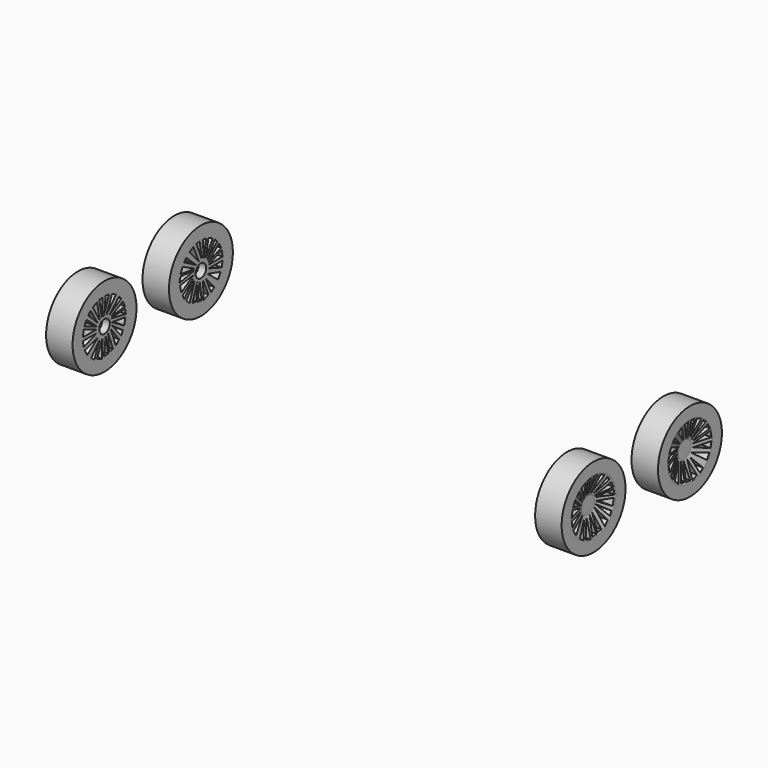
from build123d import *

# Parameters (mm, degrees)
F3_DEPTH = 54.356
F5_START = -2.0828
F4_R     = 1.016
F5_DEPTH = 5.588


# Not quite as in the source:
# - a feature names something its author has since deleted; it is built from what else it names


with BuildPart() as f1:
    # F0 (on Top) → F1 (revolve)
    with BuildSketch(Plane.XY):
        Polygon((-38.7761598104, 10.5307940394), (-38.7761598104, 9.2558898032), (-35.5391725898, 9.2558898032), (-35.5391725898, 15.3969740495), (-39.609067142, 15.3969740495), (-39.609067142, 13.5389780626), align=None)
    revolve(axis=Axis((-37.1576662001, 9.2558898032, 0), (1, 0, 0)))

    # F2 (on Right) → F3 (cut)
    with BuildSketch(Plane.YZ):
        Polygon((10.4703787739, -0.9244092506), (12.5581930749, -2.5232885566), (13.0646565989, -1.6865519105), align=None)
        Polygon((10.7676169888, -0.3009043154), (13.2498589973, -1.1950938976), (13.4170880637, -0.3009043154), align=None)
        Polygon((10.7827322258, 0.2167291751), (13.4224200405, 0.2167291751), (13.2498589973, 1.1950938976), align=None)
        Polygon((10.6890620408, 0.55644517), (13.1332652272, 1.5257193069), (12.7097717953, 2.3165763491), align=None)
        Polygon((11.9163488444, 3.1771167458), (10.4901476553, 0.8995587363), (12.3804111502, 2.7352948513), align=None)
        Polygon((11.4917309209, 3.4794998925), (10.6890620408, 3.8635174401), (10.1889797433, 1.1895302548), align=None)
        Polygon((9.647954578, 4.082242185), (9.7795484241, 1.3955574327), (10.2642306786, 3.9871991361), align=None)
        Polygon((8.386955188, 3.9871991361), (9.4131707997, 1.4628515054), (9.0197490168, 4.082242185), align=None)
        Polygon((7.0658904336, 3.4087700224), (8.8881551707, 1.3955574327), (7.823212836, 3.8054345011), align=None)
        Polygon((6.0489947183, 2.4439876807), (8.386955188, 1.1178608331), (6.4443791376, 2.9007429328), align=None)
        Polygon((5.3209666594, 1.1178608331), (8.0941571054, 0.7806299389), (5.7344314769, 1.9512906421), align=None)
        Polygon((5.156467886, 0), (7.978641554, 0.55644517), (5.3209666594, 0.8124744198), align=None)
        Polygon((5.4919943851, -1.4154481401), (7.8688514455, 0), (5.2583602836, -0.3920851117), align=None)
        Polygon((6.0489947183, -2.5315452176), (7.9222940422, -0.3920851117), (5.7344314769, -1.9512906421), align=None)
        Polygon((7.0658904336, -3.5198394674), (8.0941571054, -0.7806299389), (6.4443791376, -2.9007429328), align=None)
        Polygon((8.386955188, -3.7943273253), (8.5564610454, -1.2417284927), (7.6257726915, -3.7209981969), align=None)
        Polygon((9.4131707997, -4.0348388196), (9.0197490168, -1.4154481401), (8.5564610454, -3.952306996), align=None)
        Polygon((10.6991987211, -3.7943273253), (9.647954578, -1.4154481401), (9.7795484241, -4.1681900535), align=None)
        Polygon((11.8202538041, -3.2528705592), (10.1889797433, -1.4154481401), (11.2078192072, -3.7209981969), align=None)
    extrude(amount=-F3_DEPTH, mode=Mode.SUBTRACT)

    # F4 (on face) → F5 (cut)
    with BuildSketch(Plane(origin=(-38.7761598104, 0, 0), x_dir=(0, -1, 0), z_dir=(-1, 0, 0)).offset(F5_START)):
        with Locations((-9.2558898032, 0)):
            Circle(F4_R)
    extrude(amount=-F5_DEPTH, mode=Mode.SUBTRACT)


with BuildPart() as f6_1:
    # F6: instance of F1
    add(f1.part.mirror(Plane.XZ))


with BuildPart() as f7_1:
    # F7: instance of F1
    add(f1.part.mirror(Plane.YZ))


with BuildPart() as f7_2:
    # F7: instance of F6_1
    add(f6_1.part.mirror(Plane.YZ))


solid = Compound([f1.part, f6_1.part, f7_1.part, f7_2.part])
